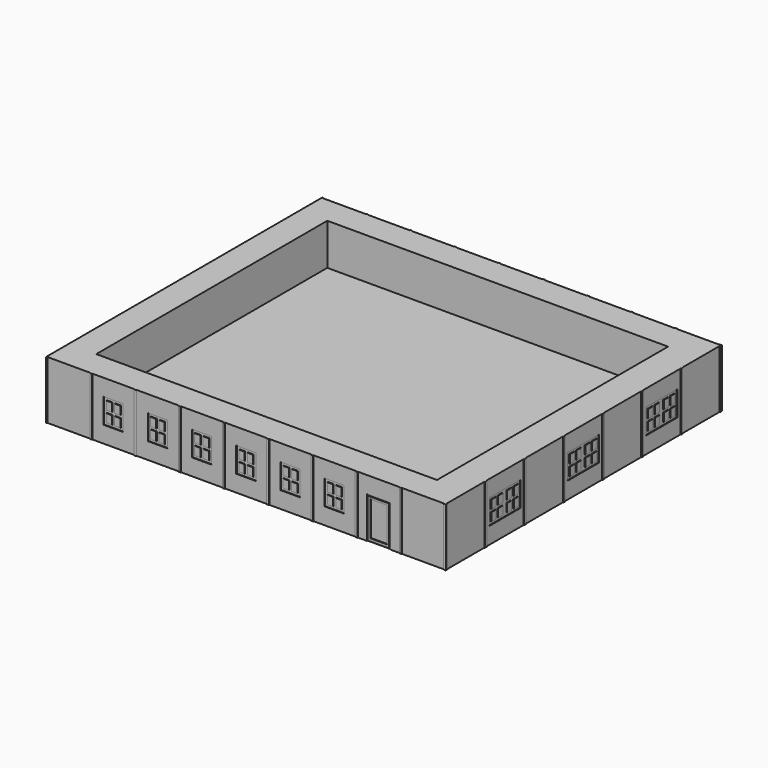
from build123d import *

# Parameters (mm, degrees)
F0_W      = 288.9
F0_H      = 249
F1_DEPTH  = 42
F2_W      = 246.6267556638
F2_H      = 209
F3_DEPTH  = 30
F4_W      = 1.6
F4_H      = 42
F4_W_2    = 0.8
F7_DEPTH  = 0.4
F5_W      = 1.6
F5_H      = 42
F8_DEPTH  = 0.4
F6_W      = 1.6
F6_H      = 42
F6_W_2    = 0.8
F9_DEPTH  = 0.4
F10_W     = 17
F10_H     = 30
F10_W_2   = 15
F10_H_2   = 28
F10_W_3   = 12
F10_H_3   = 25
F11_DEPTH = 0.5
F14_W     = 14.1428571429
F14_H     = 18
F14_W_2   = 4.1785714286
F14_H_2   = 6.1071428571
F13_W     = 14.1428571429
F13_H     = 18
F13_W_2   = 4.1785714286
F13_H_2   = 6.1071428571
F12_W     = 14.1428571429
F12_H     = 18
F12_W_2   = 4.1785714286
F12_H_2   = 6.1071428571
F15_DEPTH = 0.5
F16_W     = 14.1428571429
F16_H     = 18
F16_W_2   = 4.1785714286
F16_H_2   = 6.1071428571
F17_DEPTH = 0.5
F18_W     = 14.1428571429
F18_H     = 18
F18_W_2   = 4.1785714286
F18_H_2   = 6.1071428571
F19_DEPTH = 0.5


# Not quite as in the source:
# - a feature names something its author has since deleted; it is built from what else it names


with BuildPart() as f1:
    # F0 (on Top) → F1 (new body)
    with BuildSketch(Plane.XY):
        with Locations((144.45, -16.3575997149)):
            Rectangle(F0_W, F0_H)
    extrude(amount=F1_DEPTH)

    # F2 (on face) → F3 (cut)
    with BuildSketch(Plane.XY.offset(42)):
        with Locations((143.3133778319, -16.3575997149)):
            Rectangle(F2_W, F2_H)
    extrude(amount=-F3_DEPTH, mode=Mode.SUBTRACT)

    # F4 (on face) → F7 (join)
    with BuildSketch(Plane.XZ.offset(140.8575997149)):
        with Locations((288.5, 21)):
            Rectangle(F4_W, F4_H)
        with Locations((256.5, 21)):
            Rectangle(F4_W, F4_H)
        with Locations((224.5, 21)):
            Rectangle(F4_W, F4_H)
        with Locations((192.5, 21)):
            Rectangle(F4_W, F4_H)
        with Locations((160.5, 21)):
            Rectangle(F4_W, F4_H)
        with Locations((128.5, 21)):
            Rectangle(F4_W, F4_H)
        with Locations((96.5, 21)):
            Rectangle(F4_W, F4_H)
        with Locations((64.5, 21)):
            Rectangle(F4_W, F4_H)
        with Locations((32.5, 21)):
            Rectangle(F4_W, F4_H)
        with Locations((0.4, 21)):
            Rectangle(F4_W_2, F4_H)
    extrude(amount=F7_DEPTH)

    # F5 (on face) → F8 (join)
    with BuildSketch(Plane.YZ.offset(288.9)):
        with Locations((-140.4575997149, 21)):
            Rectangle(F5_W, F5_H)
        with Locations((-105.0004568577, 21)):
            Rectangle(F5_W, F5_H)
        with Locations((-69.5433140006, 21)):
            Rectangle(F5_W, F5_H)
        with Locations((-34.0861711434, 21)):
            Rectangle(F5_W, F5_H)
        with Locations((1.3709717137, 21)):
            Rectangle(F5_W, F5_H)
        with Locations((36.8281145709, 21)):
            Rectangle(F5_W, F5_H)
        with Locations((72.285257428, 21)):
            Rectangle(F5_W, F5_H)
        with Locations((107.7424002851, 21)):
            Rectangle(F5_W, F5_H)
    extrude(amount=F8_DEPTH)

    # F6 (on face) → F9 (join)
    with BuildSketch(Plane(origin=(0, 108.1424002851, 0), x_dir=(-1, 0, 0), z_dir=(0, 1, 0))):
        with Locations((-288.5, 21)):
            Rectangle(F6_W, F6_H)
        with Locations((-256.5, 21)):
            Rectangle(F6_W, F6_H)
        with Locations((-224.5, 21)):
            Rectangle(F6_W, F6_H)
        with Locations((-192.5, 21)):
            Rectangle(F6_W, F6_H)
        with Locations((-160.5, 21)):
            Rectangle(F6_W, F6_H)
        with Locations((-128.5, 21)):
            Rectangle(F6_W, F6_H)
        with Locations((-96.5, 21)):
            Rectangle(F6_W, F6_H)
        with Locations((-64.5, 21)):
            Rectangle(F6_W, F6_H)
        with Locations((-32.5, 21)):
            Rectangle(F6_W, F6_H)
        with Locations((-0.4, 21)):
            Rectangle(F6_W_2, F6_H)
    extrude(amount=F9_DEPTH)

    # F10 (on face) → F11 (cut)
    with BuildSketch(Plane.XZ.offset(140.8575997149)):
        with Locations((240.5, 15)):
            Rectangle(F10_W, F10_H)
        with Locations((240.5, 15)):
            Rectangle(F10_W_2, F10_H_2, mode=Mode.SUBTRACT)
        with Locations((240.5, 15)):
            Rectangle(F10_W_3, F10_H_3)
    extrude(amount=-F11_DEPTH, mode=Mode.SUBTRACT)

    # F14 (on face) + F13 (on face) + F12 (on face) → F15 (cut)
    with BuildSketch(Plane.YZ.offset(288.9)):
        with Locations((47.4850431423, 21)):
            Rectangle(F14_W, F14_H)
        with Locations((44.4314717137, 16.9821428571)):
            Rectangle(F14_W_2, F14_H_2, mode=Mode.SUBTRACT)
        with Locations((50.5386145709, 16.9821428571)):
            Rectangle(F14_W_2, F14_H_2, mode=Mode.SUBTRACT)
        with Locations((44.4314717137, 25.0178571429)):
            Rectangle(F14_W_2, F14_H_2, mode=Mode.SUBTRACT)
        with Locations((50.5386145709, 25.0178571429)):
            Rectangle(F14_W_2, F14_H_2, mode=Mode.SUBTRACT)
        with Locations((61.6279002851, 21)):
            Rectangle(F14_W, F14_H)
        with Locations((58.5743288566, 16.9821428571)):
            Rectangle(F14_W_2, F14_H_2, mode=Mode.SUBTRACT)
        with Locations((64.6814717137, 16.9821428571)):
            Rectangle(F14_W_2, F14_H_2, mode=Mode.SUBTRACT)
        with Locations((58.5743288566, 25.0178571429)):
            Rectangle(F14_W_2, F14_H_2, mode=Mode.SUBTRACT)
        with Locations((64.6814717137, 25.0178571429)):
            Rectangle(F14_W_2, F14_H_2, mode=Mode.SUBTRACT)
    with BuildSketch(Plane.YZ.offset(288.9)):
        with Locations((-23.429242572, 21)):
            Rectangle(F13_W, F13_H)
        with Locations((-26.4828140006, 16.9821428571)):
            Rectangle(F13_W_2, F13_H_2, mode=Mode.SUBTRACT)
        with Locations((-20.3756711434, 16.9821428571)):
            Rectangle(F13_W_2, F13_H_2, mode=Mode.SUBTRACT)
        with Locations((-26.4828140006, 25.0178571429)):
            Rectangle(F13_W_2, F13_H_2, mode=Mode.SUBTRACT)
        with Locations((-20.3756711434, 25.0178571429)):
            Rectangle(F13_W_2, F13_H_2, mode=Mode.SUBTRACT)
        with Locations((-9.2863854291, 21)):
            Rectangle(F13_W, F13_H)
        with Locations((-12.3399568577, 16.9821428571)):
            Rectangle(F13_W_2, F13_H_2, mode=Mode.SUBTRACT)
        with Locations((-6.2328140006, 16.9821428571)):
            Rectangle(F13_W_2, F13_H_2, mode=Mode.SUBTRACT)
        with Locations((-12.3399568577, 25.0178571429)):
            Rectangle(F13_W_2, F13_H_2, mode=Mode.SUBTRACT)
        with Locations((-6.2328140006, 25.0178571429)):
            Rectangle(F13_W_2, F13_H_2, mode=Mode.SUBTRACT)
    with BuildSketch(Plane.YZ.offset(288.9)):
        with Locations((-94.3435282863, 21)):
            Rectangle(F12_W, F12_H)
        with Locations((-97.3970997149, 16.9821428571)):
            Rectangle(F12_W_2, F12_H_2, mode=Mode.SUBTRACT)
        with Locations((-91.2899568577, 16.9821428571)):
            Rectangle(F12_W_2, F12_H_2, mode=Mode.SUBTRACT)
        with Locations((-97.3970997149, 25.0178571429)):
            Rectangle(F12_W_2, F12_H_2, mode=Mode.SUBTRACT)
        with Locations((-91.2899568577, 25.0178571429)):
            Rectangle(F12_W_2, F12_H_2, mode=Mode.SUBTRACT)
        with Locations((-80.2006711434, 21)):
            Rectangle(F12_W, F12_H)
        with Locations((-83.254242572, 16.9821428571)):
            Rectangle(F12_W_2, F12_H_2, mode=Mode.SUBTRACT)
        with Locations((-77.1470997149, 16.9821428571)):
            Rectangle(F12_W_2, F12_H_2, mode=Mode.SUBTRACT)
        with Locations((-83.254242572, 25.0178571429)):
            Rectangle(F12_W_2, F12_H_2, mode=Mode.SUBTRACT)
        with Locations((-77.1470997149, 25.0178571429)):
            Rectangle(F12_W_2, F12_H_2, mode=Mode.SUBTRACT)
    extrude(amount=-F15_DEPTH, mode=Mode.SUBTRACT)

    # F16 (on face) → F17 (cut)
    with BuildSketch(Plane.XZ.offset(140.8575997149)):
        with Locations((48.3714285714, 21)):
            Rectangle(F16_W, F16_H)
        with Locations((45.3178571429, 16.9821428571)):
            Rectangle(F16_W_2, F16_H_2, mode=Mode.SUBTRACT)
        with Locations((51.425, 16.9821428571)):
            Rectangle(F16_W_2, F16_H_2, mode=Mode.SUBTRACT)
        with Locations((45.3178571429, 25.0178571429)):
            Rectangle(F16_W_2, F16_H_2, mode=Mode.SUBTRACT)
        with Locations((51.425, 25.0178571429)):
            Rectangle(F16_W_2, F16_H_2, mode=Mode.SUBTRACT)
        with Locations((80.3714285714, 21)):
            Rectangle(F16_W, F16_H)
        with Locations((77.3178571429, 16.9821428571)):
            Rectangle(F16_W_2, F16_H_2, mode=Mode.SUBTRACT)
        with Locations((83.425, 16.9821428571)):
            Rectangle(F16_W_2, F16_H_2, mode=Mode.SUBTRACT)
        with Locations((77.3178571429, 25.0178571429)):
            Rectangle(F16_W_2, F16_H_2, mode=Mode.SUBTRACT)
        with Locations((83.425, 25.0178571429)):
            Rectangle(F16_W_2, F16_H_2, mode=Mode.SUBTRACT)
        with Locations((112.3714285714, 21)):
            Rectangle(F16_W, F16_H)
        with Locations((109.3178571429, 16.9821428571)):
            Rectangle(F16_W_2, F16_H_2, mode=Mode.SUBTRACT)
        with Locations((115.425, 16.9821428571)):
            Rectangle(F16_W_2, F16_H_2, mode=Mode.SUBTRACT)
        with Locations((109.3178571429, 25.0178571429)):
            Rectangle(F16_W_2, F16_H_2, mode=Mode.SUBTRACT)
        with Locations((115.425, 25.0178571429)):
            Rectangle(F16_W_2, F16_H_2, mode=Mode.SUBTRACT)
        with Locations((144.3714285714, 21)):
            Rectangle(F16_W, F16_H)
        with Locations((141.3178571429, 16.9821428571)):
            Rectangle(F16_W_2, F16_H_2, mode=Mode.SUBTRACT)
        with Locations((147.425, 16.9821428571)):
            Rectangle(F16_W_2, F16_H_2, mode=Mode.SUBTRACT)
        with Locations((141.3178571429, 25.0178571429)):
            Rectangle(F16_W_2, F16_H_2, mode=Mode.SUBTRACT)
        with Locations((147.425, 25.0178571429)):
            Rectangle(F16_W_2, F16_H_2, mode=Mode.SUBTRACT)
        with Locations((176.3714285714, 21)):
            Rectangle(F16_W, F16_H)
        with Locations((173.3178571429, 16.9821428571)):
            Rectangle(F16_W_2, F16_H_2, mode=Mode.SUBTRACT)
        with Locations((179.425, 16.9821428571)):
            Rectangle(F16_W_2, F16_H_2, mode=Mode.SUBTRACT)
        with Locations((173.3178571429, 25.0178571429)):
            Rectangle(F16_W_2, F16_H_2, mode=Mode.SUBTRACT)
        with Locations((179.425, 25.0178571429)):
            Rectangle(F16_W_2, F16_H_2, mode=Mode.SUBTRACT)
        Polygon((215.4428571429, 30), (201.3, 30), (201.3, 12), (215.4428571429, 12), (215.4428571429, 13.5066565126), align=None)
        with Locations((205.3178571429, 16.9821428571)):
            Rectangle(F16_W_2, F16_H_2, mode=Mode.SUBTRACT)
        with Locations((211.425, 16.9821428571)):
            Rectangle(F16_W_2, F16_H_2, mode=Mode.SUBTRACT)
        with Locations((205.3178571429, 25.0178571429)):
            Rectangle(F16_W_2, F16_H_2, mode=Mode.SUBTRACT)
        with Locations((211.425, 25.0178571429)):
            Rectangle(F16_W_2, F16_H_2, mode=Mode.SUBTRACT)
    extrude(amount=-F17_DEPTH, mode=Mode.SUBTRACT)

    # F18 (on face) → F19 (cut)
    with BuildSketch(Plane(origin=(0, 108.1424002851, 0), x_dir=(-1, 0, 0), z_dir=(0, 1, 0))):
        with Locations((-208.6285714286, 21)):
            Rectangle(F18_W, F18_H)
        with Locations((-211.6821428571, 16.9821428571)):
            Rectangle(F18_W_2, F18_H_2, mode=Mode.SUBTRACT)
        with Locations((-205.575, 16.9821428571)):
            Rectangle(F18_W_2, F18_H_2, mode=Mode.SUBTRACT)
        with Locations((-211.6821428571, 25.0178571429)):
            Rectangle(F18_W_2, F18_H_2, mode=Mode.SUBTRACT)
        with Locations((-205.575, 25.0178571429)):
            Rectangle(F18_W_2, F18_H_2, mode=Mode.SUBTRACT)
        with Locations((-176.6285714286, 21)):
            Rectangle(F18_W, F18_H)
        with Locations((-179.6821428571, 16.9821428571)):
            Rectangle(F18_W_2, F18_H_2, mode=Mode.SUBTRACT)
        with Locations((-173.575, 16.9821428571)):
            Rectangle(F18_W_2, F18_H_2, mode=Mode.SUBTRACT)
        with Locations((-179.6821428571, 25.0178571429)):
            Rectangle(F18_W_2, F18_H_2, mode=Mode.SUBTRACT)
        with Locations((-173.575, 25.0178571429)):
            Rectangle(F18_W_2, F18_H_2, mode=Mode.SUBTRACT)
        Polygon((-137.5571428571, 30), (-151.7, 30), (-151.7, 12), (-137.5571428571, 12), (-137.5571428571, 12.1485680193), align=None)
        with Locations((-147.6821428571, 16.9821428571)):
            Rectangle(F18_W_2, F18_H_2, mode=Mode.SUBTRACT)
        with Locations((-141.575, 16.9821428571)):
            Rectangle(F18_W_2, F18_H_2, mode=Mode.SUBTRACT)
        with Locations((-147.6821428571, 25.0178571429)):
            Rectangle(F18_W_2, F18_H_2, mode=Mode.SUBTRACT)
        with Locations((-141.575, 25.0178571429)):
            Rectangle(F18_W_2, F18_H_2, mode=Mode.SUBTRACT)
        Polygon((-105.5571428571, 30), (-119.7, 30), (-119.7, 12), (-105.5571428571, 12), (-105.5571428571, 13.2916826606), align=None)
        with Locations((-115.6821428571, 16.9821428571)):
            Rectangle(F18_W_2, F18_H_2, mode=Mode.SUBTRACT)
        with Locations((-109.575, 16.9821428571)):
            Rectangle(F18_W_2, F18_H_2, mode=Mode.SUBTRACT)
        with Locations((-115.6821428571, 25.0178571429)):
            Rectangle(F18_W_2, F18_H_2, mode=Mode.SUBTRACT)
        with Locations((-109.575, 25.0178571429)):
            Rectangle(F18_W_2, F18_H_2, mode=Mode.SUBTRACT)
        Polygon((-73.5571428571, 30), (-87.7, 30), (-87.7, 12), (-73.5571428571, 12), (-73.5571428571, 13.5203055888), align=None)
        with Locations((-83.6821428571, 16.9821428571)):
            Rectangle(F18_W_2, F18_H_2, mode=Mode.SUBTRACT)
        with Locations((-77.575, 16.9821428571)):
            Rectangle(F18_W_2, F18_H_2, mode=Mode.SUBTRACT)
        with Locations((-83.6821428571, 25.0178571429)):
            Rectangle(F18_W_2, F18_H_2, mode=Mode.SUBTRACT)
        with Locations((-77.575, 25.0178571429)):
            Rectangle(F18_W_2, F18_H_2, mode=Mode.SUBTRACT)
    extrude(amount=-F19_DEPTH, mode=Mode.SUBTRACT)


solid = f1.part
